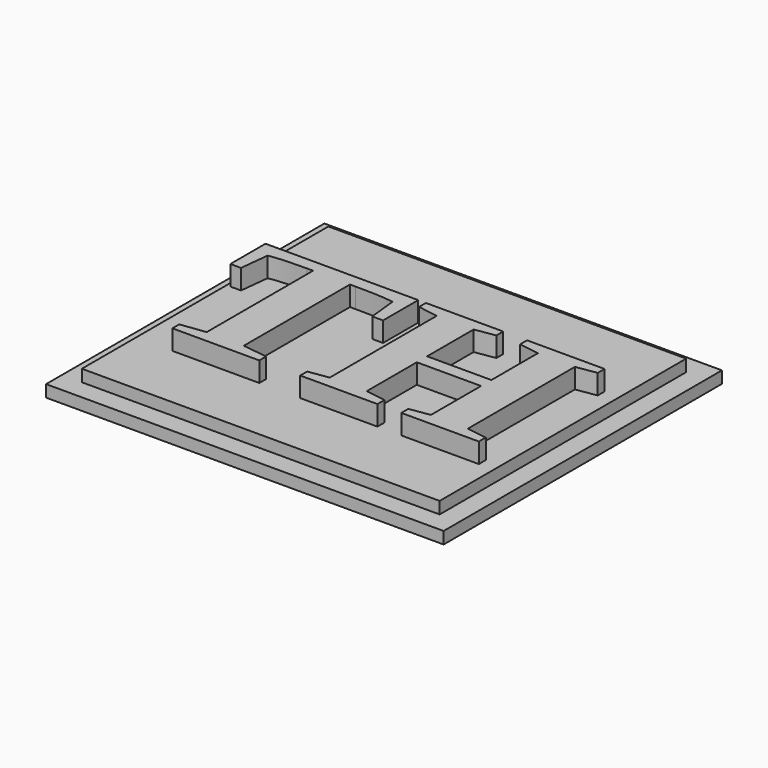
from build123d import *

# Parameters (mm, degrees)
F0_W         = 40
F0_H         = 35
F1_DEPTH     = 1.2
F2_W         = 36
F2_H         = 31
F3_DEPTH     = 1.2
F4_TEXT_SIZE = 24.1484121161
F5_DEPTH     = 2


# Not quite as in the source:
# - Text() gives the source's letters only with a copy of the font that has no kerning and outlines rounded to 1/6400 em; it was checked with that copy


with BuildPart() as f1:
    # F0 (on Top) → F1 (new body)
    with BuildSketch(Plane.XY):
        with Locations((20, 17.5)):
            Rectangle(F0_W, F0_H)
    extrude(amount=F1_DEPTH)

    # F2 (on face) → F3 (join)
    with BuildSketch(Plane.XY.offset(1.2)):
        with Locations((20, 17.5)):
            Rectangle(F2_W, F2_H)
    extrude(amount=F3_DEPTH)

    # F4 (on face) → F5 (join)
    with BuildSketch(Plane.XY.offset(2.4)):
        with Locations((2, 8.8131432764)):
            Text('TH', F4_TEXT_SIZE, font='Tinos', font_style=FontStyle.BOLD, text_align=(TextAlign.LEFT, TextAlign.BOTTOM))
    extrude(amount=F5_DEPTH)


solid = f1.part
